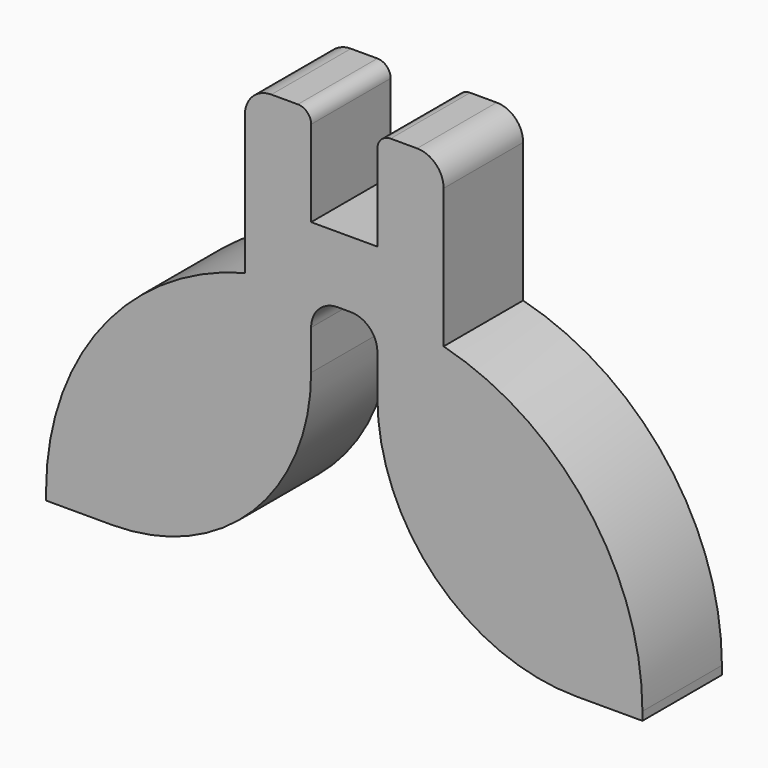
from build123d import *

# Parameters (mm, degrees)
F0_W        = 6.35
F0_H        = 12.7
F1_DEPTH    = 19.05
F2_R        = 2.54
F3_R        = 38.1
F4_T1_DEPTH = 264.9844424842
F5_R        = 5.08
F6_R        = 5.08


# Not quite as in the source:
# - a fillet or chamfer that OpenCascade refuses, or shapes differently, is made with other operations: its cross-section is extruded or revolved along the edge and cut away or added


with BuildPart() as f1:
    # F0 (on Front) → F1 (new body)
    with BuildSketch(Plane.XZ):
        Polygon((-6.35, -50.8), (-6.35, 0), (-19.05, 0), (-57.15, 0), (-57.15, -50.8), align=None)
        Polygon((-19.05, 0), (-6.35, 0), (-6.35, 12.7), (-6.35, 31.75), (-19.05, 31.75), align=None)
        with Locations((-3.175, 6.35)):
            Rectangle(F0_W, F0_H)
        with Locations((3.175, 6.35)):
            Rectangle(F0_W, F0_H)
        Polygon((6.35, 12.7), (6.35, 0), (19.05, 0), (19.05, 31.75), (6.35, 31.75), align=None)
        Polygon((19.05, 0), (6.35, 0), (6.35, -50.8), (57.15, -50.8), (57.15, 0), align=None)
    extrude(amount=F1_DEPTH)

    # F2
    f2_edges = [f1.edges().sort_by_distance(p)[0] for p in [
        (6.35, -9.525, 31.75),
        (-6.35, -9.525, 31.75),
    ]]
    fillet(f2_edges, radius=F2_R)

    # F3
    f3_edges = [f1.edges().sort_by_distance(p)[0] for p in [
        (6.35, -9.525, -50.8),
        (-6.35, -9.525, -50.8),
    ]]
    fillet(f3_edges, radius=F3_R)

    # F4: fillet of radius 50.8 on 2 edges, made by hand

    # F4_s2 → F4_t1 (cut)
    with BuildSketch(Plane.XZ.offset(-122.9672212421)):
        with BuildLine():
            ThreePointArc((-57.15, -49.1868884968), (-46.5109262841, -18.0783687635), (-19.05, 0))
            Line((-19.05, 0), (-57.15, 0))
            Line((-57.15, 0), (-57.15, -49.1868884968))
        make_face()
        with BuildLine():
            ThreePointArc((57.15, -49.1868884968), (46.5109262841, -18.0783687635), (19.05, 0))
            Line((19.05, 0), (57.15, 0))
            Line((57.15, 0), (57.15, -49.1868884968))
        make_face()
    extrude(amount=F4_T1_DEPTH, mode=Mode.SUBTRACT)

    # F5
    f5_edges = [f1.edges().sort_by_distance(p)[0] for p in [
        (-19.05, -9.525, 31.75),
        (19.05, -9.525, 31.75),
    ]]
    fillet(f5_edges, radius=F5_R)

    # F6
    f6_edges = [f1.edges().sort_by_distance(p)[0] for p in [
        (6.35, -9.525, 0),
        (-6.35, -9.525, 0),
    ]]
    fillet(f6_edges, radius=F6_R)


solid = f1.part
